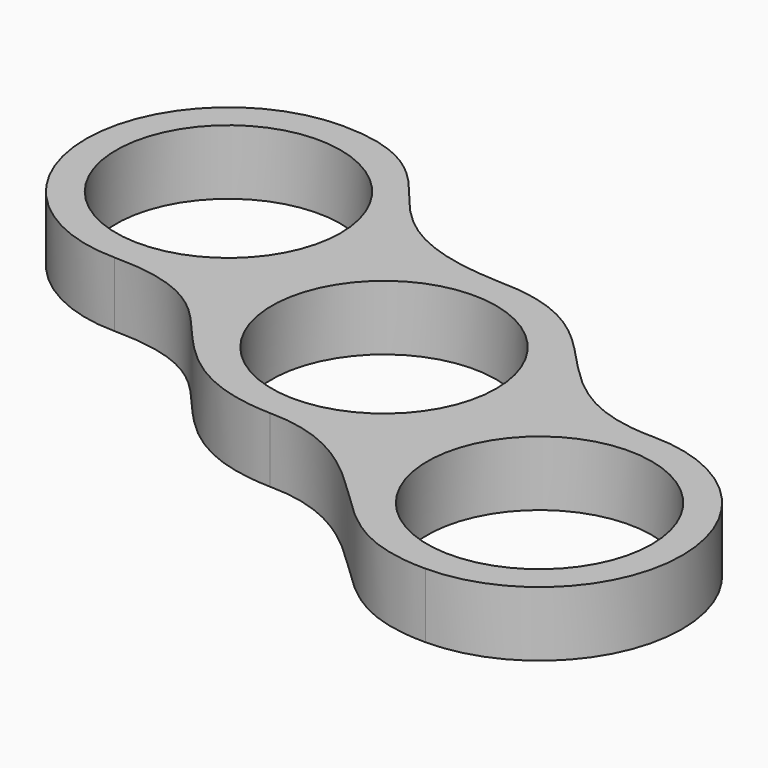
from build123d import *

# Parameters (mm, degrees)
F0_R     = 10.9982
F1_DEPTH = 6.35


with BuildPart() as f1:
    # F0 (on Top) → F1 (new body)
    with BuildSketch(Plane.XY):
        with BuildLine():
            add(Edge.make_bspline(
                [(0, -13.97), (5.7787014373, -13.97), (13.1291277882, -20.32), (18.7630429864, -26.67), (25.4, -26.67)],
                knots=[0, 0, 0, 0, 0.5, 1, 1, 1, 1], degree=3))
            ThreePointArc((25.4, -26.67), (39.37, -12.7), (25.4, 1.27))
            add(Edge.make_bspline(
                [(0, 13.97), (6.853028044, 13.97), (12.6391638998, 7.6416874466), (18.8445616513, 1.27), (25.4, 1.27)],
                knots=[0, 0, 0, 0, 0.500853834, 1, 1, 1, 1], degree=3))
            add(Edge.make_bspline(
                [(-25.4, 26.67), (-17.5831354201, 26.67), (-13.6102278083, 17.9003816405), (-6.4407057817, 14.2221620935), (0, 13.97)],
                knots=[0, 0, 0, 0, 0.5099402335, 1, 1, 1, 1], degree=3))
            ThreePointArc((-25.4, 26.67), (-39.37, 12.7), (-25.4, -1.27))
            add(Edge.make_bspline(
                [(-25.4, -1.27), (-17.5831354201, -1.27), (-13.269427077, -7.7050659785), (-6.678010426, -13.799868043), (0, -13.97)],
                knots=[0, 0, 0, 0, 0.5, 1, 1, 1, 1], degree=3))
        make_face()
        Circle(F0_R, mode=Mode.SUBTRACT)
        with Locations((25.4, -12.7)):
            Circle(F0_R, mode=Mode.SUBTRACT)
        with Locations((-25.4, 12.7)):
            Circle(F0_R, mode=Mode.SUBTRACT)
    extrude(amount=F1_DEPTH)


solid = f1.part
